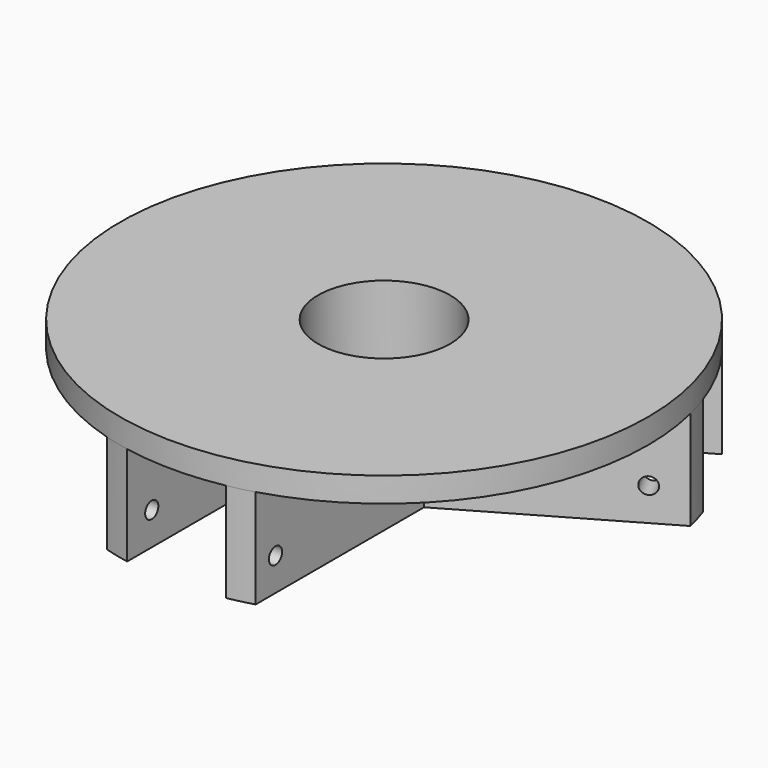
from build123d import *

# Parameters (mm, degrees)
F3_DEPTH = 38.1
F4_R     = 3.175
F5_DEPTH = 76.2
F6_R     = 3.175
F7_DEPTH = 76.2
F8_R     = 3.175
F9_DEPTH = 76.2


with BuildPart() as f1:
    # F0 (on Front) → F1 (revolve)
    with BuildSketch(Plane.XZ):
        Polygon((101.6, 0), (25.4, 0), (25.4, -47.625), (31.75, -47.625), (31.75, -9.525), (101.6, -9.525), align=None)
    revolve(axis=Axis((0, 0, -4.0980735794), (0, 0, -1)))

    # F2 (on face) → F3 (join)
    with BuildSketch(Plane(origin=(0, 0, -9.525), x_dir=(1, 0, 0), z_dir=(0, 0, -1))):
        with BuildLine():
            Line((-28.575, 13.8395041457), (-28.575, 16.4977839421))
            Line((-28.575, 16.4977839421), (-98.7239970333, -24.0027583784))
            ThreePointArc((-98.7239970333, -24.0027583784), (-97.4517043144, -28.7354367675), (-95.952675689, -33.4012578824))
            Line((-95.952675689, -33.4012578824), (-31.5220452561, 3.7977839421))
            ThreePointArc((-31.5220452561, 3.7977839421), (-30.4651070619, 8.9409032938), (-28.575, 13.8395041457))
        make_face()
        with BuildLine():
            Line((-12.4720452561, -29.1977839421), (-76.902675689, -66.3968257666))
            ThreePointArc((-76.902675689, -66.3968257666), (-73.6114703867, -70.0279331946), (-70.1489970333, -73.4961102047))
            Line((-70.1489970333, -73.4961102047), (0, -32.9955678842))
            Line((0, -32.9955678842), (-2.302137834, -31.666427986))
            ThreePointArc((-2.302137834, -31.666427986), (-7.4895041457, -30.8540082915), (-12.4720452561, -29.1977839421))
        make_face()
        with BuildLine():
            ThreePointArc((2.302137834, -31.666427986), (0, -31.75), (-2.302137834, -31.666427986))
            Line((-2.302137834, -31.666427986), (0, -32.9955678842))
            Line((0, -32.9955678842), (2.302137834, -31.666427986))
        make_face()
        with BuildLine():
            ThreePointArc((70.1489970333, -73.4961102047), (73.6114703867, -70.0279331946), (76.902675689, -66.3968257666))
            Line((76.902675689, -66.3968257666), (12.4720452561, -29.1977839421))
            ThreePointArc((12.4720452561, -29.1977839421), (7.4895041457, -30.8540082915), (2.302137834, -31.666427986))
            Line((2.302137834, -31.666427986), (0, -32.9955678842))
            Line((0, -32.9955678842), (70.1489970333, -73.4961102047))
        make_face()
        with BuildLine():
            Line((98.7239970333, -24.0027583784), (28.575, 16.4977839421))
            Line((28.575, 16.4977839421), (28.575, 13.8395041457))
            ThreePointArc((28.575, 13.8395041457), (30.4651070619, 8.9409032938), (31.5220452561, 3.7977839421))
            Line((31.5220452561, 3.7977839421), (95.952675689, -33.4012578824))
            ThreePointArc((95.952675689, -33.4012578824), (97.4517043144, -28.7354367675), (98.7239970333, -24.0027583784))
        make_face()
        with BuildLine():
            ThreePointArc((-28.575, 13.8395041457), (-27.4963065702, 15.875), (-26.272862166, 17.8269238403))
            Line((-26.272862166, 17.8269238403), (-28.575, 16.4977839421))
            Line((-28.575, 16.4977839421), (-28.575, 13.8395041457))
        make_face()
        with BuildLine():
            Line((-19.05, 25.4), (-19.05, 99.7980836489))
            ThreePointArc((-19.05, 99.7980836489), (-23.8402339277, 98.7633699621), (-28.575, 97.4988685832))
            Line((-28.575, 97.4988685832), (-28.575, 16.4977839421))
            Line((-28.575, 16.4977839421), (-26.272862166, 17.8269238403))
            ThreePointArc((-26.272862166, 17.8269238403), (-22.9756029161, 21.9131049977), (-19.05, 25.4))
        make_face()
        with BuildLine():
            Line((28.575, 16.4977839421), (26.272862166, 17.8269238403))
            ThreePointArc((26.272862166, 17.8269238403), (27.4963065702, 15.875), (28.575, 13.8395041457))
            Line((28.575, 13.8395041457), (28.575, 16.4977839421))
        make_face()
        with BuildLine():
            ThreePointArc((28.575, 97.4988685832), (23.8402339277, 98.7633699621), (19.05, 99.7980836489))
            Line((19.05, 99.7980836489), (19.05, 25.4))
            ThreePointArc((19.05, 25.4), (22.9756029161, 21.9131049977), (26.272862166, 17.8269238403))
            Line((26.272862166, 17.8269238403), (28.575, 16.4977839421))
            Line((28.575, 16.4977839421), (28.575, 97.4988685832))
        make_face()
    extrude(amount=F3_DEPTH)

    # F4 (on face) → F5 (cut)
    with BuildSketch(Plane.YZ.offset(28.575)):
        with Locations((-87.9738685832, -34.925)):
            Circle(F4_R)
    extrude(amount=-F5_DEPTH, mode=Mode.SUBTRACT)

    # F6 (on face) → F7 (cut)
    with BuildSketch(Plane(origin=(14.2875, -24.7466759131, 0), x_dir=(0.8660254038, 0.5, 0), z_dir=(0.5, -0.8660254038, 0))):
        with Locations((84.7988685832, -34.925)):
            Circle(F6_R)
    extrude(amount=-F7_DEPTH, mode=Mode.SUBTRACT)

    # F8 (on face) → F9 (cut)
    with BuildSketch(Plane(origin=(-14.2875, -24.7466759131, 0), x_dir=(0.8660254038, -0.5, 0), z_dir=(-0.5, -0.8660254038, 0))):
        with Locations((-84.7988685832, -34.925)):
            Circle(F8_R)
    extrude(amount=-F9_DEPTH, mode=Mode.SUBTRACT)


solid = f1.part
